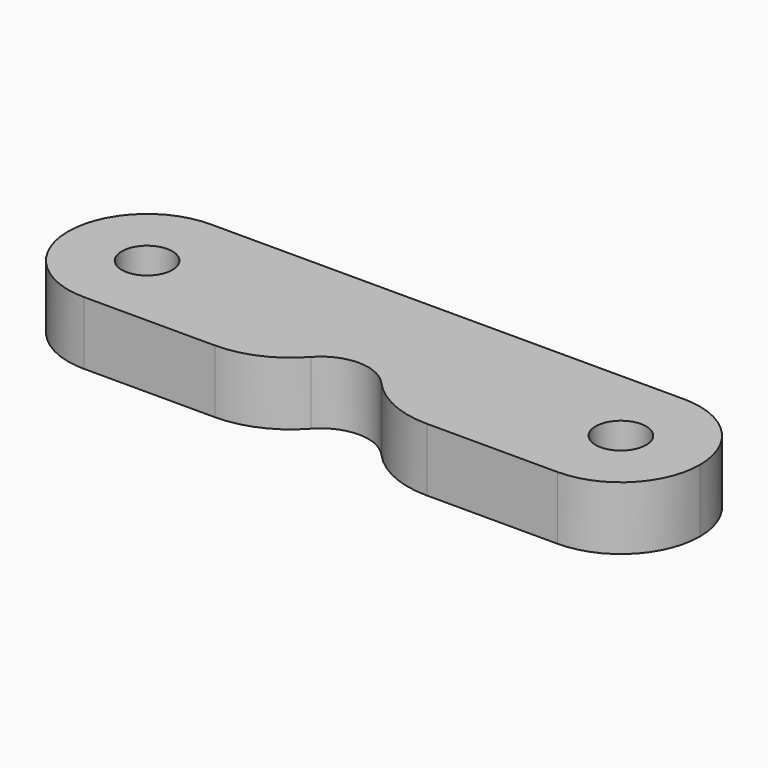
from build123d import *

# Parameters (mm, degrees)
F0_W     = 40
F0_H     = 10
F0_R     = 1.6
F1_DEPTH = 4
F2_R     = 1.5
F3_DEPTH = 1.5
F4_R     = 4.99999
F5_R     = 3
F6_DEPTH = 25
F7_R     = 6


# Not quite as in the source:
# - a fillet or chamfer is up to 0.001 mm smaller than in the source, because OpenCascade refuses the exact size


with BuildPart() as f1:
    # F0 (on Top) → F1 (new body)
    with BuildSketch(Plane.XY):
        Rectangle(F0_W, F0_H)
        with Locations((-15, 0)):
            Circle(F0_R, mode=Mode.SUBTRACT)
        with Locations((15, 0)):
            Circle(F0_R, mode=Mode.SUBTRACT)
    extrude(amount=F1_DEPTH)

    # F2 (on face) → F3 (cut)
    with BuildSketch(Plane(origin=(0, 0, 0), x_dir=(1, 0, 0), z_dir=(0, 0, -1))):
        with Locations((-7, 0)):
            Circle(F2_R)
        with Locations((7, 0)):
            Circle(F2_R)
    extrude(amount=-F3_DEPTH, mode=Mode.SUBTRACT)

    # F4 (radius 5 in the source; OpenCascade refuses exactly that, so slightly less here)
    f4_edges = [f1.edges().sort_by_distance(p)[0] for p in [
        (-20, -5, 2),
        (-20, 5, 2),
        (20, 5, 2),
        (20, -5, 2),
    ]]
    fillet(f4_edges, radius=F4_R)

    # F5 (on face) → F6 (cut)
    with BuildSketch(Plane.XY.offset(4)):
        with Locations((0, -5)):
            Circle(F5_R)
    extrude(amount=-F6_DEPTH, mode=Mode.SUBTRACT)

    # F7
    f7_edges = [f1.edges().sort_by_distance(p)[0] for p in [
        (3, -5, 2),
        (-3, -5, 2),
    ]]
    fillet(f7_edges, radius=F7_R)


solid = f1.part
